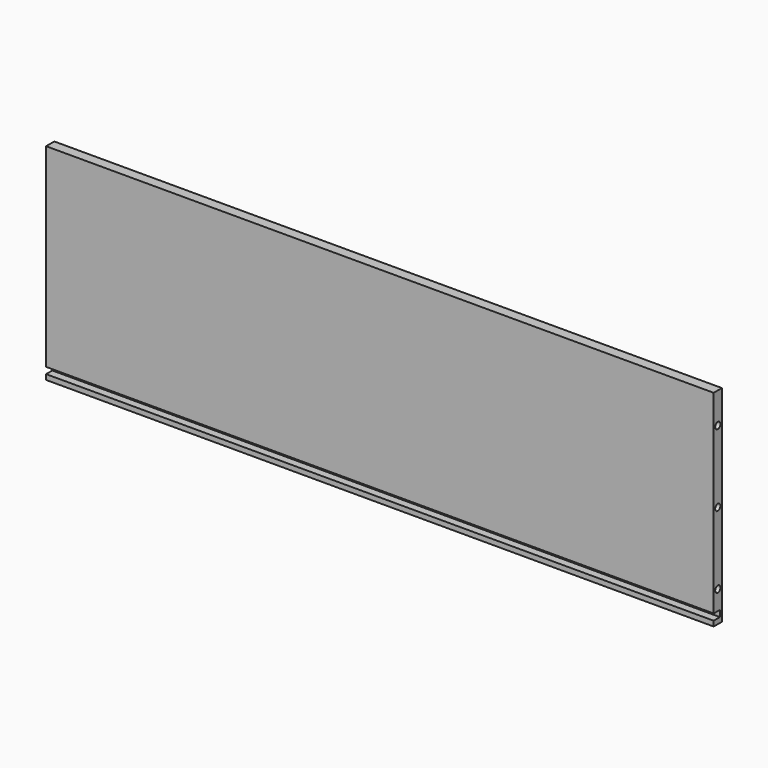
from build123d import *

# Parameters (mm, degrees)
F0_W     = 823.976
F0_H     = 254
F1_DEPTH = 12.7
F2_W     = 823.976
F2_H     = 7.874
F3_DEPTH = 9.652
F5_D     = 8.001
F5_DEPTH = 25.4
F5_TIP   = 2.4037429064
F7_D     = 8.001
F7_DEPTH = 25.4
F7_TIP   = 2.4037429064


with BuildPart() as f1:
    # F0 (on Front) → F1 (new body)
    with BuildSketch(Plane.XZ):
        Rectangle(F0_W, F0_H)
    extrude(amount=F1_DEPTH)

    # F2 (on face) → F3 (cut)
    with BuildSketch(Plane.XZ.offset(12.7)):
        with Locations((0, -116.713)):
            Rectangle(F2_W, F2_H)
    extrude(amount=-F3_DEPTH, mode=Mode.SUBTRACT)

    # F5
    with Locations(Plane(origin=(-411.988, 0, 0), x_dir=(0, -1, 0), z_dir=(-1, 0, 0))):
        with Locations((6.35, 88.9), (6.35, 0), (6.35, -88.9)):
            Hole(F5_D / 2, depth=F5_DEPTH)
            with Locations((0, 0, -(F5_DEPTH + F5_TIP / 2))):  # 118° drill point
                Cone(0, F5_D / 2, F5_TIP, mode=Mode.SUBTRACT)

    # F7
    with Locations(Plane.YZ.offset(411.988)):
        with Locations((-6.35, 88.9), (-6.35, 0), (-6.35, -88.9)):
            Hole(F7_D / 2, depth=F7_DEPTH)
            with Locations((0, 0, -(F7_DEPTH + F7_TIP / 2))):  # 118° drill point
                Cone(0, F7_D / 2, F7_TIP, mode=Mode.SUBTRACT)


solid = f1.part
